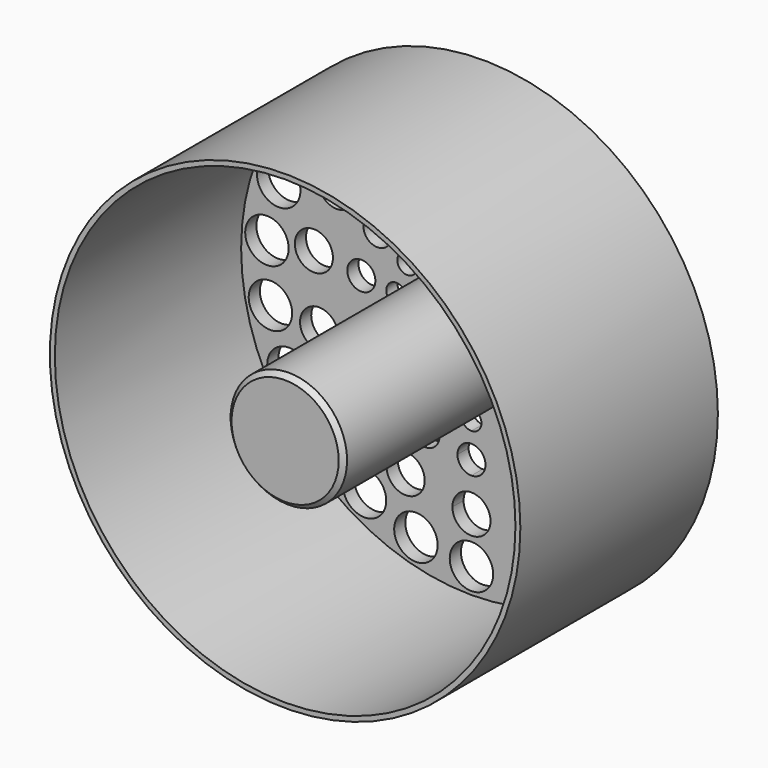
from build123d import *

# Parameters (mm, degrees)
F0_R             = 50.5
F1_DEPTH         = 3
F2_R             = 50.5
F2_R_2           = 49.4440908639
F3_DEPTH         = 50
F4_R             = 12.5
F5_DEPTH         = 50
F6_SIZE          = 1
F9_R             = 4.6632476683
F10_DEPTH        = 53.001
F10_COPIES_COUNT = 10
F10_COPIES_ANGLE = 141.4287
F11_R            = 4.0917082841
F11_R_2          = 3.0111553801
F11_R_3          = 2.1424193095
F12_DEPTH        = 53.001


# Not quite as in the source:
# - a pattern or mirror of a feature is missing from the dataset's text; its kind, count and spacing are read off the source's solid


with BuildPart() as f1:
    # F0 (on Front) → F1 (new body)
    with BuildSketch(Plane.XZ):
        Circle(F0_R)
    extrude(amount=F1_DEPTH)

    # F2 (on face) → F3 (join)
    with BuildSketch(Plane.XZ.offset(3)):
        Circle(F2_R)
        Circle(F2_R_2, mode=Mode.SUBTRACT)
    extrude(amount=F3_DEPTH)

    # F4 (on face) → F5 (join)
    with BuildSketch(Plane.XZ.offset(3)):
        Circle(F4_R)
    extrude(amount=F5_DEPTH)

    # F6
    f6_edges = [f1.edges().sort_by_distance(p)[0] for p in [
        (-12.5, -53, 0),
    ]]
    chamfer(f6_edges, length=F6_SIZE)

    # F9 (on face) → F10 (cut, through all)
    with BuildSketch(Plane(origin=(0, 0, 0), x_dir=(-1, 0, 0), z_dir=(0, 1, 0))):
        with Locations((0, -44.030174613)):
            Circle(F9_R)
    f10 = extrude(amount=-F10_DEPTH, mode=Mode.SUBTRACT)

    # F10_copies: F10 ×10 about axis
    f10_copies_axis = Axis((0, 0, 0), (0, 1, 0))
    for i in range(1, F10_COPIES_COUNT):
        add(f10.rotate(f10_copies_axis, i * F10_COPIES_ANGLE / (F10_COPIES_COUNT - 1)), mode=Mode.SUBTRACT)

    # F10_copies1: F10 across plane
    add(f10.mirror(Plane(origin=(0, 0, 0), x_dir=(0.9801724878, 0, 0.1981461432), z_dir=(-0.1981461432, 0, 0.9801724878))), mode=Mode.SUBTRACT)

    # F10_copies2: F10 across plane
    add(f10.mirror(Plane(origin=(0, 0, 0), x_dir=(0.9980579158, 0, 0.0622928302), z_dir=(-0.0622928302, 0, 0.9980579158))), mode=Mode.SUBTRACT)

    # F10_copies3: F10 across plane
    add(f10.mirror(Plane(origin=(0, 0, 0), x_dir=(0.9972037972, 0, -0.0747300936), z_dir=(0.0747300936, 0, 0.9972037972))), mode=Mode.SUBTRACT)

    # F10_copies4: F10 across plane
    add(f10.mirror(Plane(origin=(0, 0, 0), x_dir=(0.9776261689, 0, -0.2103498843), z_dir=(0.2103498843, 0, 0.9776261689))), mode=Mode.SUBTRACT)

    # F10_copies5: F10 across plane
    add(f10.mirror(Plane(origin=(0, 0, 0), x_dir=(0.9396926208, 0, -0.3420201433), z_dir=(0.3420201433, 0, 0.9396926208))), mode=Mode.SUBTRACT)

    # F11 (on face) → F12 (cut, through all)
    with BuildSketch(Plane(origin=(0, 0, 0), x_dir=(-1, 0, 0), z_dir=(0, 1, 0))):
        with Locations((-9.1548590747, 32.8874919017)):
            Circle(F11_R)
        with Locations((-6.3979976493, 22.98387055)):
            Circle(F11_R_2)
        with Locations((-4.3693644676, 15.6963026268)):
            Circle(F11_R_3)
        with Locations((-10.4730058489, 12.4812423457)):
            Circle(F11_R_3)
        with Locations((-15.3354720805, 18.2761039461)):
            Circle(F11_R_2)
        with Locations((-21.9434412824, 26.1511749822)):
            Circle(F11_R)
        with Locations((5.2749524196, 33.7279327151)):
            Circle(F11_R)
        with Locations((3.686472168, 23.5712240313)):
            Circle(F11_R_2)
        with Locations((2.5175908752, 16.0974220976)):
            Circle(F11_R_3)
        with Locations((18.7591014711, 28.5218281367)):
            Circle(F11_R)
        with Locations((13.1100529385, 19.9328671126)):
            Circle(F11_R_2)
        with Locations((8.9532073342, 13.6126904187)):
            Circle(F11_R_3)
        with Locations((28.8802291505, 18.2024979735)):
            Circle(F11_R)
        with Locations((20.1833405306, 12.7210630218)):
            Circle(F11_R_2)
        with Locations((13.7837454444, 8.6875556704)):
            Circle(F11_R_3)
        with Locations((33.8238792195, 4.6199310394)):
            Circle(F11_R)
        with Locations((25.7207452383, -22.4464213773)):
            Circle(F11_R)
        with Locations((17.9752922715, -15.6869865537)):
            Circle(F11_R_2)
        with Locations((32.7037831717, -9.7908699573)):
            Circle(F11_R)
        with Locations((22.855483208, -6.8424824959)):
            Circle(F11_R_2)
        with Locations((14.1266433863, -31.0779104011)):
            Circle(F11_R)
        with BuildLine():
            ThreePointArc((0, -30.0462261622), (-2.8932746743, -37.0312091207), (4.0917082841, -34.1379344463))
            ThreePointArc((4.0917082841, -34.1379344463), (2.8932746743, -31.244659772), (0, -30.0462261622))
        make_face()
        with BuildLine():
            ThreePointArc((0, -20.8466039317), (-3.0111553801, -23.8577593118), (0, -26.8689146919))
            Line((0, -26.8689146919), (0, -20.8466039317))
        make_face()
        with BuildLine():
            Line((0, -20.8466039317), (0, -26.8689146919))
            ThreePointArc((0, -26.8689146919), (2.1292083885, -25.9869677003), (3.0111553801, -23.8577593118))
            ThreePointArc((3.0111553801, -23.8577593118), (2.1292083885, -21.7285509233), (0, -20.8466039317))
        make_face()
        with Locations((9.8725966659, -21.7192199319)):
            Circle(F11_R_2)
        with BuildLine():
            ThreePointArc((0, -14.1506854285), (-2.1424193095, -16.293104738), (0, -18.4355240475))
            Line((0, -18.4355240475), (0, -14.1506854285))
        make_face()
        with BuildLine():
            Line((0, -14.1506854285), (0, -18.4355240475))
            ThreePointArc((0, -18.4355240475), (1.5149192219, -17.8080239599), (2.1424193095, -16.293104738))
            ThreePointArc((2.1424193095, -16.293104738), (1.5149192219, -14.7781855161), (0, -14.1506854285))
        make_face()
        with Locations((6.7422614761, -14.8326387468)):
            Circle(F11_R_3)
        with Locations((12.2758099722, -10.7130645256)):
            Circle(F11_R_3)
        with Locations((15.6086234621, -4.6729151098)):
            Circle(F11_R_3)
        with Locations((23.6382775495, 3.2287015768)):
            Circle(F11_R_2)
        with Locations((16.1432147465, 2.2049670412)):
            Circle(F11_R_3)
    extrude(amount=-F12_DEPTH, mode=Mode.SUBTRACT)


solid = f1.part
